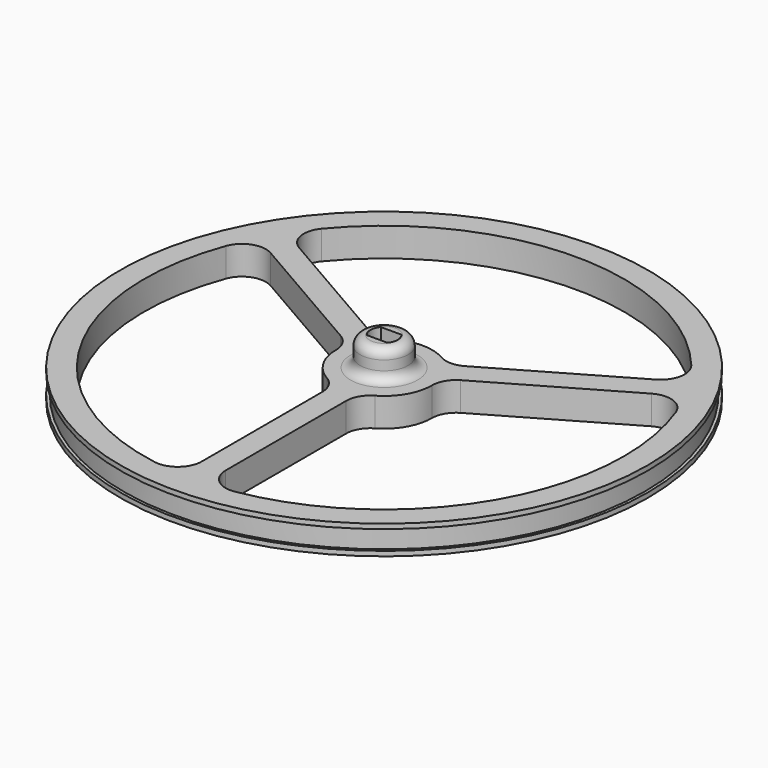
from build123d import *

# Parameters (mm, degrees)
F0_R         = 55
F1_DEPTH     = 6
F2_R         = 5
F3_DEPTH     = 6
F5_DEPTH     = 8
F7_R         = 55
F7_R_2       = 54.4
F8_DEPTH     = 4
F10_DEPTH    = 25
F11_R        = 5
F12_T1_DEPTH = 6
F13_R        = 2


# Not quite as in the source:
# - a fillet or chamfer that OpenCascade refuses, or shapes differently, is made with other operations: its cross-section is extruded or revolved along the edge and cut away or added


with BuildPart() as f1:
    # F0 (on Top) → F1 (new body)
    with BuildSketch(Plane.XY):
        Circle(F0_R)
    extrude(amount=F1_DEPTH)

    # F2 (on face) → F3 (join)
    with BuildSketch(Plane.XY.offset(6)):
        Circle(F2_R)
    extrude(amount=F3_DEPTH)

    # F4 (on face) → F5 (cut)
    with BuildSketch(Plane.XY.offset(12)):
        with BuildLine():
            Line((2.1498313887, 1.825), (-2.1498313887, 1.825))
            ThreePointArc((-2.1498313887, 1.825), (-2.82, 0), (-2.1498313887, -1.825))
            Line((-2.1498313887, -1.825), (2.1498313887, -1.825))
            ThreePointArc((2.1498313887, -1.825), (2.82, 0), (2.1498313887, 1.825))
        make_face()
    extrude(amount=-F5_DEPTH, mode=Mode.SUBTRACT)

    # F7 (on offset) → F8 (cut)
    with BuildSketch(Plane.XY.offset(1)):
        Circle(F7_R)
        Circle(F7_R_2, mode=Mode.SUBTRACT)
    extrude(amount=F8_DEPTH, mode=Mode.SUBTRACT)

    # F9 (on face) → F10 (cut)
    with BuildSketch(Plane.XY.offset(6)):
        with BuildLine():
            Line((7.1352549156, 7.0062926922), (41.9971112805, 27.1337948489))
            ThreePointArc((41.9971112805, 27.1337948489), (0, 50.0000017881), (-41.9971112805, 27.1337948489))
            Line((-41.9971112805, 27.1337948489), (-7.1352549156, 7.0062926922))
            ThreePointArc((-7.1352549156, 7.0062926922), (0, 10), (7.1352549156, 7.0062926922))
        make_face()
        with BuildLine():
            ThreePointArc((2.5, -49.937462679), (36.2284431303, -34.460123145), (50.0000017881, 0))
            ThreePointArc((50.0000017881, 0), (48.6048136629, 11.729120496), (44.4971112805, 22.80366783))
            Line((44.4971112805, 22.80366783), (9.6352549156, 2.6761656733))
            ThreePointArc((9.6352549156, 2.6761656733), (9.9083941473, 1.3504537837), (10, 0))
            ThreePointArc((10, 0), (7.9056941504, -6.123724357), (2.5, -9.6824583655))
            Line((2.5, -9.6824583655), (2.5, -49.937462679))
        make_face()
        with BuildLine():
            ThreePointArc((-44.4971112805, 22.80366783), (-43.3012717378, -25.0000008941), (-2.5, -49.937462679))
            Line((-2.5, -49.937462679), (-2.5, -9.6824583655))
            ThreePointArc((-2.5, -9.6824583655), (-8.6602540378, -5), (-9.6352549156, 2.6761656733))
            Line((-9.6352549156, 2.6761656733), (-44.4971112805, 22.80366783))
        make_face()
    extrude(amount=-F10_DEPTH, mode=Mode.SUBTRACT)

    # F11
    f11_edges = [f1.edges().sort_by_distance(p)[0] for p in [
        (-44.497111, 22.803668, 3),
        (-41.997111, 27.133795, 3),
        (41.997111, 27.133795, 3),
        (44.497111, 22.803668, 3),
        (2.5, -49.937463, 3),
        (-2.5, -49.937463, 3),
    ]]
    fillet(f11_edges, radius=F11_R)

    # F12: fillet of radius 5 on 6 edges, made by hand

    # F12_s2 → F12_t1 (join)
    with BuildSketch(Plane.XY):
        with BuildLine():
            ThreePointArc((-12.5, 4.3301270189), (-10.6698729811, 2.5), (-10, 0))
            ThreePointArc((-10, 0), (-9.9083941473, 1.3504537837), (-9.6352549156, 2.6761656733))
            Line((-9.6352549156, 2.6761656733), (-12.5, 4.3301270189))
        make_face()
        with BuildLine():
            ThreePointArc((-5, -8.6602540378), (-3.1698729811, -10.4903810568), (-2.5, -12.9903810568))
            Line((-2.5, -12.9903810568), (-2.5, -9.6824583655))
            ThreePointArc((-2.5, -9.6824583655), (-3.7846697903, -9.2561479341), (-5, -8.6602540378))
        make_face()
        with BuildLine():
            ThreePointArc((2.5, -12.9903810568), (3.1698729811, -10.4903810568), (5, -8.6602540378))
            ThreePointArc((5, -8.6602540378), (3.7846697903, -9.2561479341), (2.5, -9.6824583655))
            Line((2.5, -9.6824583655), (2.5, -12.9903810568))
        make_face()
        with BuildLine():
            ThreePointArc((12.5, 4.3301270189), (10.6698729811, 2.5), (10, 0))
            ThreePointArc((10, 0), (9.9083941473, 1.3504537837), (9.6352549156, 2.6761656733))
            Line((9.6352549156, 2.6761656733), (12.5, 4.3301270189))
        make_face()
        with BuildLine():
            ThreePointArc((10, 8.6602540378), (7.5, 7.9903810568), (5, 8.6602540378))
            ThreePointArc((5, 8.6602540378), (6.123724357, 7.9056941504), (7.1352549156, 7.0062926922))
            Line((7.1352549156, 7.0062926922), (10, 8.6602540378))
        make_face()
        with BuildLine():
            ThreePointArc((-10, 8.6602540378), (-7.5, 7.9903810568), (-5, 8.6602540378))
            ThreePointArc((-5, 8.6602540378), (-6.123724357, 7.9056941504), (-7.1352549156, 7.0062926922))
            Line((-7.1352549156, 7.0062926922), (-10, 8.6602540378))
        make_face()
    extrude(amount=F12_T1_DEPTH)

    # F13
    f13_edges = [f1.edges().sort_by_distance(p)[0] for p in [
        (-5, 0, 6),
        (-5, 0, 12),
    ]]
    fillet(f13_edges, radius=F13_R)


solid = f1.part
